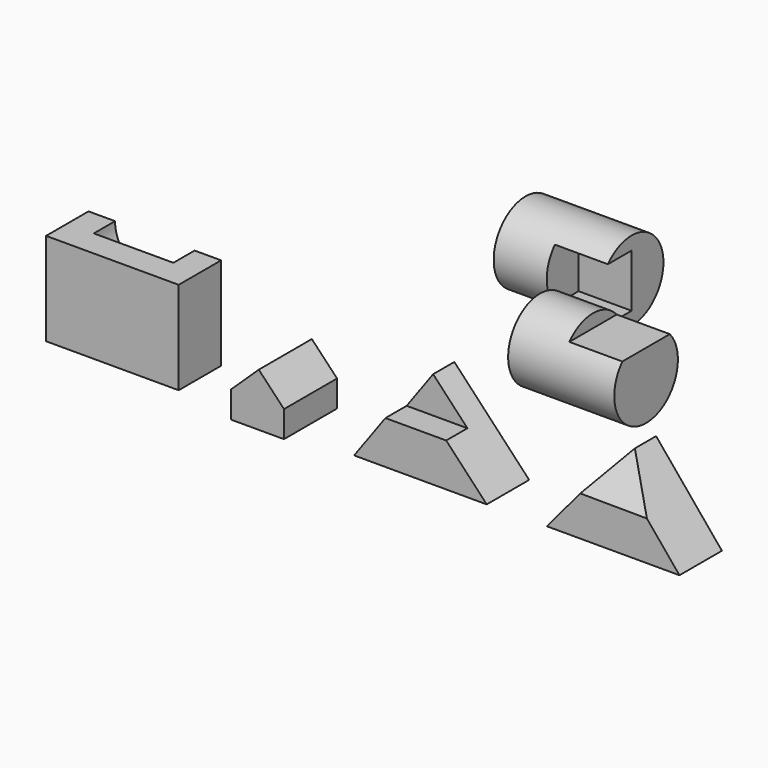
from build123d import *

# Parameters (mm, degrees)
F1_DEPTH  = 101.6
F3_DEPTH  = 50.8
F5_DEPTH  = 101.6
F9_DEPTH  = 177.8
F11_DEPTH = 127
F16_R     = 76.2
F17_DEPTH = 203.2
F19_DEPTH = 101.6
F20_R     = 76.2
F21_DEPTH = 203.2
F23_DEPTH = 101.6
F25_DEPTH = 101.6
F27_DEPTH = 50.8


# Not quite as in the source:
# - the program builds the solid bodies; features that only make, move or delete a surface that nothing else refers to are left out


with BuildPart() as f1:
    # F0 (on Front) → F1 (new body)
    with BuildSketch(Plane.XZ):
        Polygon((0, 151.7990483895), (-110.6943220668, -0.6009516105), (143.3056779332, -0.6009516105), align=None)
    extrude(amount=F1_DEPTH)

    # F2 (on face) → F3 (cut)
    with BuildSketch(Plane.XZ.offset(101.6)):
        Polygon((-50.7436143692, 81.9370474714), (0, 81.9370474714), (65.6930538277, 81.9370474714), (0, 151.7990483895), align=None)
    extrude(amount=-F3_DEPTH, mode=Mode.SUBTRACT)


with BuildPart() as f5:
    # F4 (on Front) → F5 (new body)
    with BuildSketch(Plane.XZ):
        Polygon((386.4619200636, 152.4), (258.5280877834, 0), (512.5280877834, 0), align=None)
    extrude(amount=F5_DEPTH)

    # F8 (on 3pt) → F9 (cut, symmetric)
    with BuildSketch(Plane(origin=(385.5136131508, 0, -2.362237903), x_dir=(0, 1, 0), z_dir=(0.9999812273, 0, -0.0061273934))):
        Polygon((-50.8, 154.765143255), (-101.6, 154.765143255), (-101.6, 78.1746232731), align=None)
    extrude(amount=F9_DEPTH, both=True, mode=Mode.SUBTRACT)


with BuildPart() as f11:
    # F10 (on Front) → F11 (new body)
    with BuildSketch(Plane.XZ):
        Polygon((-326.3838480476, 0), (-224.7838480476, 0), (-224.6583398959, 50.8), (-272.99527684, 101.6), (-326.3838480476, 50.8), align=None)
    extrude(amount=F11_DEPTH)


with BuildPart() as f17:
    # F16 (on Right) → F17 (new body)
    with BuildSketch(Plane.YZ):
        with Locations((205.0628811121, 107.5141951442)):
            Circle(F16_R)
    extrude(amount=F17_DEPTH)

    # F18 (on face) → F19 (cut)
    with BuildSketch(Plane.YZ.offset(203.2)):
        with BuildLine():
            ThreePointArc((205.0628811121, 183.7141951442), (173.9543613788, 177.0749599473), (148.2667544836, 158.3141951442))
            Line((148.2667544836, 158.3141951442), (205.0628811121, 158.3141951442))
            Line((205.0628811121, 158.3141951442), (205.0628811121, 183.7141951442))
        make_face()
        with BuildLine():
            Line((205.0628811121, 183.7141951442), (205.0628811121, 158.3141951442))
            Line((205.0628811121, 158.3141951442), (261.8590077406, 158.3141951442))
            ThreePointArc((261.8590077406, 158.3141951442), (236.1714008454, 177.0749599473), (205.0628811121, 183.7141951442))
        make_face()
    extrude(amount=-F19_DEPTH, mode=Mode.SUBTRACT)


with BuildPart() as f21:
    # F20 (on Right) → F21 (new body)
    with BuildSketch(Plane.YZ):
        with Locations((424.4354069233, 116.2917613983)):
            Circle(F20_R)
    extrude(amount=-F21_DEPTH)

    # F22 (on face) → F23 (cut)
    with BuildSketch(Plane.YZ):
        with BuildLine():
            Line((424.4354069233, 65.4917613983), (424.4354069233, 116.2917613983))
            Line((424.4354069233, 116.2917613983), (424.4354069233, 167.0917613983))
            Line((424.4354069233, 167.0917613983), (367.6392802948, 167.0917613983))
            ThreePointArc((367.6392802948, 167.0917613983), (348.2354069233, 116.2917613983), (367.6392802948, 65.4917613983))
            Line((367.6392802948, 65.4917613983), (424.4354069233, 65.4917613983))
        make_face()
    extrude(amount=-F23_DEPTH, mode=Mode.SUBTRACT)


with BuildPart() as f25:
    # F24 (on Front) → F25 (new body)
    with BuildSketch(Plane.XZ):
        with BuildLine():
            Line((-700.7503095217, 0), (-446.7503095217, 0))
            Line((-446.7503095217, 0), (-446.7503095217, 177.8))
            Line((-446.7503095217, 177.8), (-497.5503095217, 177.8))
            ThreePointArc((-497.5503095217, 177.8), (-573.7503095217, 101.6), (-649.9503095217, 177.8))
            Line((-649.9503095217, 177.8), (-700.7503095217, 177.8))
            Line((-700.7503095217, 177.8), (-700.7503095217, 0))
        make_face()
    extrude(amount=F25_DEPTH)

    # F26 (on face) → F27 (join)
    with BuildSketch(Plane.XZ.offset(101.6)):
        with BuildLine():
            ThreePointArc((-649.9503095217, 177.8), (-573.7503095217, 101.6), (-497.5503095217, 177.8))
            Line((-497.5503095217, 177.8), (-649.9503095217, 177.8))
        make_face()
    extrude(amount=-F27_DEPTH)


solid = Compound([f1.part, f5.part, f11.part, f17.part, f21.part, f25.part])
